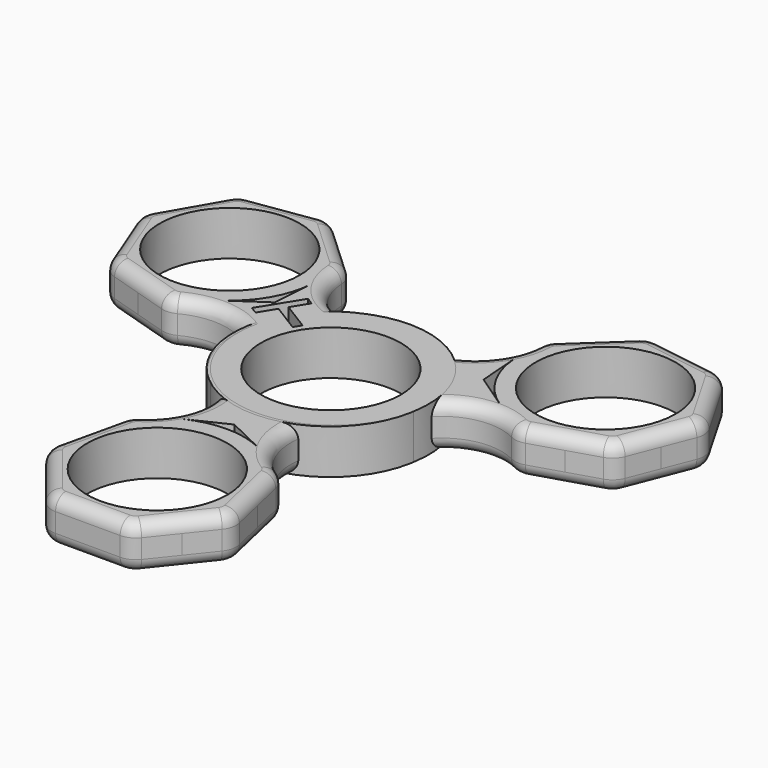
from build123d import *

# Parameters (mm, degrees)
F1_DEPTH       = 7
F2_R           = 10.9982
F3_DEPTH       = 7.001
F5_COUNT       = 3
F6_R           = 3.1
F6_2_R         = 3.1
F6_3_R         = 3.1
F7_T1_DEPTH    = 10.2686412317
F7_T3_DEPTH    = 10.25929714
F7_T5_DEPTH    = 10.1415011295
F7_T7_DEPTH    = 10.1415011295
F7_T9_DEPTH    = 10.1415011295
F7_T12_ANGLE   = 51.4285714286
F7_T14_ANGLE   = 44.6985802325
F7_T18_ANGLE   = 95.7149736929
F7_S19_R       = 15.0569162084
F7_T20_DEPTH   = 12
F7_T22_ANGLE   = 51.4285714286
F7_T24_ANGLE   = 51.4285714286
F7_T26_ANGLE   = 51.4285714286
F7_T28_ANGLE   = 44.1929451945
F7_T32_ANGLE   = 104.4319543532
F7_S33_R       = 15.0569162084
F7_T34_DEPTH   = 13
F7_T36_ANGLE   = 44.1929451945
F7_T38_ANGLE   = 51.4285714286
F7_T40_ANGLE   = 51.4285714286
F7_T42_ANGLE   = 51.4285714286
F7_T44_ANGLE   = 51.4285714286
F7_T46_ANGLE   = 44.6985802325
F7_T50_ANGLE   = 95.7149736929
F7_S51_R       = 15.0569162084
F7_T52_DEPTH   = 12
F7_T56_ANGLE   = 104.4319543532
F7_S57_R       = 15.0569162084
F7_T58_DEPTH   = 13
F7_2_T1_DEPTH  = 10.1415011295
F7_2_T3_DEPTH  = 10.2686412317
F7_2_T5_DEPTH  = 10.1415011295
F7_2_T7_DEPTH  = 10.1415011295
F7_2_T9_DEPTH  = 10.25929714
F7_2_T12_ANGLE = 44.1929451945
F7_2_T14_ANGLE = 51.4285714286
F7_2_T16_ANGLE = 51.4285714286
F7_2_T18_ANGLE = 51.4285714286
F7_2_T20_ANGLE = 51.4285714286
F7_2_T22_ANGLE = 44.6985802325
F7_2_T26_ANGLE = 95.7149736929
F7_2_S27_R     = 15.0569162084
F7_2_T28_DEPTH = 13
F7_2_T32_ANGLE = 104.4319543532
F7_2_S33_R     = 15.0569162084
F7_2_T34_DEPTH = 12
F7_2_T36_ANGLE = 51.4285714286
F7_2_T38_ANGLE = 51.4285714286
F7_2_T40_ANGLE = 44.6985802325
F7_2_T44_ANGLE = 95.7149736929
F7_2_S45_R     = 15.0569162084
F7_2_T46_DEPTH = 13
F7_2_T48_ANGLE = 51.4285714286
F7_2_T50_ANGLE = 51.4285714286
F7_2_T52_ANGLE = 44.1929451945
F7_2_T56_ANGLE = 104.4319543532
F7_2_S57_R     = 15.0569162084
F7_2_T58_DEPTH = 12
F7_3_T1_DEPTH  = 10.25929714
F7_3_T3_DEPTH  = 10.1415011295
F7_3_T5_DEPTH  = 10.1415011295
F7_3_T7_DEPTH  = 10.1415011295
F7_3_T9_DEPTH  = 10.2686412317
F7_3_T12_ANGLE = 44.1929451945
F7_3_T14_ANGLE = 51.4285714286
F7_3_T16_ANGLE = 51.4285714286
F7_3_T18_ANGLE = 51.4285714286
F7_3_T20_ANGLE = 51.4285714286
F7_3_T22_ANGLE = 44.6985802325
F7_3_T26_ANGLE = 95.7149736929
F7_3_S27_R     = 15.0569162084
F7_3_T28_DEPTH = 13
F7_3_T32_ANGLE = 104.4319543532
F7_3_S33_R     = 15.0569162084
F7_3_T34_DEPTH = 13
F7_3_T36_ANGLE = 51.4285714286
F7_3_T38_ANGLE = 51.4285714286
F7_3_T40_ANGLE = 44.1929451945
F7_3_T44_ANGLE = 104.4319543532
F7_3_S45_R     = 15.0569162084
F7_3_T46_DEPTH = 13
F7_3_T48_ANGLE = 51.4285714286
F7_3_T50_ANGLE = 51.4285714286
F7_3_T52_ANGLE = 44.6985802325
F7_3_T56_ANGLE = 95.7149736929
F7_3_S57_R     = 15.0569162084
F7_3_T58_DEPTH = 13
F8_R           = 10.9982
F9_DEPTH       = 7.0010001


# Not quite as in the source:
# - a fillet or chamfer that OpenCascade refuses, or shapes differently, is made with other operations: its cross-section is extruded or revolved along the edge and cut away or added
# - a feature names something its author has since deleted; it is built from what else it names


with BuildPart() as f1:
    # F0 (on Top) → F1 (new body)
    with BuildSketch(Plane.XY):
        with BuildLine():
            ThreePointArc((10.6559893288, -42.5716732307), (12.8646786322, -38.5753509396), (13.6295220444, -34.0738051109))
            ThreePointArc((13.6295220444, -34.0738051109), (13.5438224971, -32.5477830518), (13.2878015765, -31.0409515996))
            ThreePointArc((13.2878015765, -31.0409515996), (10.655989621, -25.5759373575), (5.9136281245, -21.7940301308))
            ThreePointArc((5.9136281245, -21.7940301308), (-6.034e-07, -20.4442830665), (-5.9136292117, -21.7940306543))
            ThreePointArc((-5.9136292117, -21.7940306543), (-10.655989762, -25.5759375342), (-13.2878014086, -31.0409508638))
            ThreePointArc((-13.2878014086, -31.0409508638), (-13.28780149, -37.1066590013), (-10.6559893588, -42.5716731931))
            ThreePointArc((-10.6559893588, -42.5716731931), (-5.9136279392, -46.3535801803), (-4e-10, -47.7033271552))
            ThreePointArc((-4e-10, -47.7033271552), (5.9136279171, -46.3535801909), (10.6559893288, -42.5716732307))
        make_face()
        with BuildLine():
            ThreePointArc((13.2878015765, -31.0409515996), (13.5438224971, -32.5477830518), (13.6295220444, -34.0738051109))
            ThreePointArc((13.6295220444, -34.0738051109), (12.8646786322, -38.5753509396), (10.6559893288, -42.5716732307))
            Line((10.6559893288, -42.5716732307), (14.7483469675, -37.4400190643))
            Line((14.7483469675, -37.4400190643), (13.2878015765, -31.0409515996))
        make_face()
        with BuildLine():
            ThreePointArc((5.9136281245, -21.7940301308), (10.655989621, -25.5759373575), (13.2878015765, -31.0409515996))
            Line((13.2878015765, -31.0409515996), (11.827255974, -24.6418832081))
            Line((11.827255974, -24.6418832081), (6.1794303068, -21.9220337154))
            Line((6.1794303068, -21.9220337154), (5.9136281245, -21.7940301308))
        make_face()
        with BuildLine():
            Line((6.563631883, -47.7033271552), (10.6559893288, -42.5716732307))
            ThreePointArc((10.6559893288, -42.5716732307), (5.9136279171, -46.3535801909), (-4e-10, -47.7033271552))
            Line((-4e-10, -47.7033271552), (6.563631883, -47.7033271552))
        make_face()
        with BuildLine():
            Line((0, -18.9461769209), (5.9136281245, -21.7940301308))
            Line((5.9136281245, -21.7940301308), (6.1794303068, -21.9220337154))
            ThreePointArc((6.1794303068, -21.9220337154), (4.8033446668, -17.8576663017), (4.8404350008, -13.5668250708))
            Line((4.8404350008, -13.5668250708), (6.1794303068, -13.5668250708))
            ThreePointArc((6.1794303068, -13.5668250708), (-0.1592409852, 15.0955047693), (-6.9180878725, -13.4706621833))
            Line((-6.9180878725, -13.4706621833), (-5.5738588853, -13.4706621833))
            ThreePointArc((-5.5738588853, -13.4706621833), (-5.5961038295, -18.7704883426), (-8.6417702198, -23.1078341203))
            Line((-8.6417702198, -23.1078341203), (-5.9136292117, -21.7940306543))
            Line((-5.9136292117, -21.7940306543), (0, -18.9461769209))
        make_face()
        with BuildLine():
            Line((6.1794303068, -21.9220337154), (11.827255974, -24.6418832081))
            ThreePointArc((11.827255974, -24.6418832081), (7.1362076022, -20.0565167273), (6.1794303068, -13.5668250708))
            Line((6.1794303068, -13.5668250708), (4.8404350008, -13.5668250708))
            ThreePointArc((4.8404350008, -13.5668250708), (4.8033446668, -17.8576663017), (6.1794303068, -21.9220337154))
        make_face()
        with BuildLine():
            Line((-6.563631883, -47.7033271552), (-4e-10, -47.7033271552))
            ThreePointArc((-4e-10, -47.7033271552), (-5.9136279392, -46.3535801803), (-10.6559893588, -42.5716731931))
            Line((-10.6559893588, -42.5716731931), (-6.563631883, -47.7033271552))
        make_face()
        with BuildLine():
            ThreePointArc((-13.2878014086, -31.0409508638), (-10.655989762, -25.5759375342), (-5.9136292117, -21.7940306543))
            Line((-5.9136292117, -21.7940306543), (-8.6417702198, -23.1078341203))
            Line((-8.6417702198, -23.1078341203), (-11.827255974, -24.6418832081))
            Line((-11.827255974, -24.6418832081), (-13.2878014086, -31.0409508638))
        make_face()
        with BuildLine():
            Line((-14.7483469675, -37.4400190643), (-10.6559893588, -42.5716731931))
            ThreePointArc((-10.6559893588, -42.5716731931), (-13.28780149, -37.1066590013), (-13.2878014086, -31.0409508638))
            Line((-13.2878014086, -31.0409508638), (-14.7483469675, -37.4400190643))
        make_face()
        with BuildLine():
            Line((-11.827255974, -24.6418832081), (-8.6417702198, -23.1078341203))
            ThreePointArc((-8.6417702198, -23.1078341203), (-5.5961038295, -18.7704883426), (-5.5738588853, -13.4706621833))
            Line((-5.5738588853, -13.4706621833), (-6.9180878725, -13.4706621833))
            ThreePointArc((-6.9180878725, -13.4706621833), (-7.3085566508, -19.963343537), (-11.827255974, -24.6418832081))
        make_face()
    extrude(amount=F1_DEPTH)

    # F2 (on face) → F3 (cut, through all)
    with BuildSketch(Plane.XY.offset(7)):
        Circle(F2_R)
        with Locations((0, -34.0738051109)):
            Circle(F2_R)
    extrude(amount=-F3_DEPTH, mode=Mode.SUBTRACT)


with BuildPart() as f5_1:
    # F5: instance of F1
    add(f1.part.rotate(Axis((0, 0, 10.0436238572), (0, 0, 1)), 1 * 360 / F5_COUNT))

    # F6#2
    f6_2_edges = [f5_1.edges().sort_by_distance(p)[0] for p in [
        (15.426869, 22.563646, 3.5),
        (25.049834, 31.492453, 3.5),
        (38.030477, 29.535936, 3.5),
        (44.594109, 18.167392, 3.5),
        (39.798181, 5.947566, 3.5),
        (27.254125, 2.078237, 3.5),
    ]]
    fillet(f6_2_edges, radius=F6_2_R)

    # F7#2: fillet of radius 2 on 2 edges, made by hand

    # F7_2_s2 → F7_2_t1 (cut)
    with BuildSketch(Plane(origin=(31.3565415396, -4.7262381861, 0), x_dir=(0, 0, 1), z_dir=(-0.9888308262, 0.1490422662, 0))):
        with BuildLine():
            ThreePointArc((7, 32.8741920415), (6.4142135624, 34.2884056039), (5, 34.8741920415))
            Line((5, 34.8741920415), (7, 34.8741920415))
            Line((7, 34.8741920415), (7, 32.8741920415))
        make_face()
        with BuildLine():
            ThreePointArc((0, 32.8741920415), (0.5857864376, 34.2884056039), (2, 34.8741920415))
            Line((2, 34.8741920415), (0, 34.8741920415))
            Line((0, 34.8741920415), (0, 32.8741920415))
        make_face()
    extrude(amount=F7_2_T1_DEPTH, mode=Mode.SUBTRACT)

    # F7_2_s4 → F7_2_t3 (cut)
    with BuildSketch(Plane(origin=(26.7766913665, 8.25951543, 0), x_dir=(0, 0, 1), z_dir=(0.9555728058, 0.2947551744, 0))):
        with BuildLine():
            ThreePointArc((2, 6.0473871076), (0.5857864376, 5.46160067), (0, 4.0473871076))
            Line((0, 4.0473871076), (0, 6.0473871076))
            Line((0, 6.0473871076), (2, 6.0473871076))
        make_face()
        with BuildLine():
            ThreePointArc((5, 6.0473871076), (6.4142135624, 5.46160067), (7, 4.0473871076))
            Line((7, 4.0473871076), (7, 6.0473871076))
            Line((7, 6.0473871076), (5, 6.0473871076))
        make_face()
    extrude(amount=F7_2_T3_DEPTH, mode=Mode.SUBTRACT)

    # F7_2_s6 → F7_2_t5 (cut)
    with BuildSketch(Plane(origin=(7.880122025, 20.0782234679, 0), x_dir=(0, 0, 1), z_dir=(0.3653410244, 0.9308737486, 0))):
        with BuildLine():
            ThreePointArc((0, 32.8741920415), (0.5857864376, 34.2884056039), (2, 34.8741920415))
            Line((2, 34.8741920415), (0, 34.8741920415))
            Line((0, 34.8741920415), (0, 32.8741920415))
        make_face()
        with BuildLine():
            ThreePointArc((7, 32.8741920415), (6.4142135624, 34.2884056039), (5, 34.8741920415))
            Line((5, 34.8741920415), (7, 34.8741920415))
            Line((7, 34.8741920415), (7, 32.8741920415))
        make_face()
    extrude(amount=F7_2_T5_DEPTH, mode=Mode.SUBTRACT)

    # F7_2_s8 → F7_2_t7 (cut)
    with BuildSketch(Plane(origin=(2.5353752824, -4.3913988053, 0), x_dir=(0, 0, 1), z_dir=(-0.5, 0.8660254038, 0))):
        with BuildLine():
            ThreePointArc((0, 45.7033271552), (0.5857864376, 47.1175407176), (2, 47.7033271552))
            Line((2, 47.7033271552), (0, 47.7033271552))
            Line((0, 47.7033271552), (0, 45.7033271552))
        make_face()
        with BuildLine():
            ThreePointArc((7, 45.7033271552), (6.4142135624, 47.1175407176), (5, 47.7033271552))
            Line((5, 47.7033271552), (7, 47.7033271552))
            Line((7, 47.7033271552), (7, 45.7033271552))
        make_face()
    extrude(amount=F7_2_T7_DEPTH, mode=Mode.SUBTRACT)

    # F7_2_s10 → F7_2_t9 (cut)
    with BuildSketch(Plane(origin=(28.0687425446, 26.0439870574, 0), x_dir=(0, 0, 1), z_dir=(-0.7330518718, -0.6801727378, 0))):
        with BuildLine():
            ThreePointArc((0, 4.0473871076), (0.5857864376, 5.46160067), (2, 6.0473871076))
            Line((2, 6.0473871076), (0, 6.0473871076))
            Line((0, 6.0473871076), (0, 4.0473871076))
        make_face()
        with BuildLine():
            ThreePointArc((7, 4.0473871076), (6.4142135624, 5.46160067), (5, 6.0473871076))
            Line((5, 6.0473871076), (7, 6.0473871076))
            Line((7, 6.0473871076), (7, 4.0473871076))
        make_face()
    extrude(amount=F7_2_T9_DEPTH, mode=Mode.SUBTRACT)

    # F7_2_s11 → F7_2_t12 (revolve, cut)
    with BuildSketch(Plane(origin=(26.7766913665, 8.25951543, 0), x_dir=(0, 0, 1), z_dir=(0.9555728058, 0.2947551744, 0))):
        with BuildLine():
            ThreePointArc((0, 4.0473871076), (0.5857864376, 5.46160067), (2, 6.0473871076))
            Line((2, 6.0473871076), (0, 6.0473871076))
            Line((0, 6.0473871076), (0, 4.0473871076))
        make_face()
    revolve(axis=Axis((27.6454489675, 5.4430724618, 0), (0, 0, -1)), revolution_arc=F7_2_T12_ANGLE, mode=Mode.SUBTRACT)

    # F7_2_s13 → F7_2_t14 (revolve, cut)
    with BuildSketch(Plane(origin=(36.5891256799, 11.2862505672, 0), x_dir=(0, 0, 1), z_dir=(-0.9555728058, -0.2947551744, 0))):
        with BuildLine():
            ThreePointArc((0, -4.0473871076), (0.5857864376, -5.46160067), (2, -6.0473871076))
            Line((2, -6.0473871076), (0, -6.0473871076))
            Line((0, -6.0473871076), (0, -4.0473871076))
        make_face()
    revolve(axis=Axis((37.4578832809, 8.469807599, 0), (0, 0, 1)), revolution_arc=F7_2_T14_ANGLE, mode=Mode.SUBTRACT)

    # F7_2_s15 → F7_2_t16 (revolve, cut)
    with BuildSketch(Plane(origin=(11.5852284363, 29.5186806412, 0), x_dir=(0, 0, 1), z_dir=(-0.3653410244, -0.9308737486, 0))):
        with BuildLine():
            ThreePointArc((0, -32.8741920415), (0.5857864376, -34.2884056039), (2, -34.8741920415))
            Line((2, -34.8741920415), (0, -34.8741920415))
            Line((0, -34.8741920415), (0, -32.8741920415))
        make_face()
    revolve(axis=Axis((41.1629896921, 17.9102647723, 0), (0, 0, 1)), revolution_arc=F7_2_T16_ANGLE, mode=Mode.SUBTRACT)

    # F7_2_s17 → F7_2_t18 (revolve, cut)
    with BuildSketch(Plane(origin=(-2.5353752824, 4.3913988053, 0), x_dir=(0, 0, 1), z_dir=(0.5, -0.8660254038, 0))):
        with BuildLine():
            ThreePointArc((0, -45.7033271552), (0.5857864376, -47.1175407176), (2, -47.7033271552))
            Line((2, -47.7033271552), (0, -47.7033271552))
            Line((0, -47.7033271552), (0, -45.7033271552))
        make_face()
    revolve(axis=Axis((36.0922391274, 26.6930623829, 0), (0, 0, 1)), revolution_arc=F7_2_T18_ANGLE, mode=Mode.SUBTRACT)

    # F7_2_s19 → F7_2_t20 (revolve, cut)
    with BuildSketch(Plane(origin=(21.3283125986, -3.2147258753, 0), x_dir=(0, 0, 1), z_dir=(0.9888308262, -0.1490422662, 0))):
        with BuildLine():
            ThreePointArc((0, -32.8741920415), (0.5857864376, -34.2884056039), (2, -34.8741920415))
            Line((2, -34.8741920415), (0, -34.8741920415))
            Line((0, -34.8741920415), (0, -32.8741920415))
        make_face()
    revolve(axis=Axis((26.0640101864, 28.2045746937, 0), (0, 0, 1)), revolution_arc=F7_2_T20_ANGLE, mode=Mode.SUBTRACT)

    # F7_2_s21 → F7_2_t22 (revolve, cut)
    with BuildSketch(Plane(origin=(0.9381651249, 21.9779882774, 0), x_dir=(0, 0, 1), z_dir=(-0.0426477412, -0.9990901712, 0))):
        with BuildLine():
            ThreePointArc((0, -16.5212804378), (0.5857864376, -15.1070668755), (2, -14.5212804378))
            Line((2, -14.5212804378), (0, -14.5212804378))
            Line((0, -14.5212804378), (0, -16.5212804378))
        make_face()
    revolve(axis=Axis((18.5434132142, 21.2264804704, 0), (0, 0, -1)), revolution_arc=F7_2_T22_ANGLE, mode=Mode.SUBTRACT)


with BuildPart() as f5_2:
    # F5: instance of F1
    add(f1.part.rotate(Axis((0, 0, 10.0436238572), (0, 0, 1)), 2 * 360 / F5_COUNT))

    # F6
    f6_edges = [f5_2.edges().sort_by_distance(p)[0] for p in [
        (-44.594109, 18.167392, 3.5),
        (-38.030477, 29.535936, 3.5),
        (-25.049834, 31.492453, 3.5),
        (-39.798181, 5.947566, 3.5),
        (-27.254125, 2.078237, 3.5),
        (-15.426869, 22.563646, 3.5),
    ]]
    fillet(f6_edges, radius=F6_R)

    # F7: fillet of radius 2 on 2 edges, made by hand

    # F7_s2 → F7_t1 (cut)
    with BuildSketch(Plane(origin=(-20.5412958686, 19.0595372377, 0), x_dir=(0, 0, 1), z_dir=(-0.7330518718, 0.6801727378, 0))):
        with BuildLine():
            ThreePointArc((5, 6.0473871076), (6.4142135624, 5.46160067), (7, 4.0473871076))
            Line((7, 4.0473871076), (7, 6.0473871076))
            Line((7, 6.0473871076), (5, 6.0473871076))
        make_face()
        with BuildLine():
            ThreePointArc((2, 6.0473871076), (0.5857864376, 5.46160067), (0, 4.0473871076))
            Line((0, 4.0473871076), (0, 6.0473871076))
            Line((0, 6.0473871076), (2, 6.0473871076))
        make_face()
    extrude(amount=F7_T1_DEPTH, mode=Mode.SUBTRACT)

    # F7_s4 → F7_t3 (cut)
    with BuildSketch(Plane(origin=(-36.5891256799, 11.2862505672, 0), x_dir=(0, 0, 1), z_dir=(0.9555728058, -0.2947551744, 0))):
        with BuildLine():
            ThreePointArc((0, 4.0473871076), (0.5857864376, 5.46160067), (2, 6.0473871076))
            Line((2, 6.0473871076), (0, 6.0473871076))
            Line((0, 6.0473871076), (0, 4.0473871076))
        make_face()
        with BuildLine():
            ThreePointArc((7, 4.0473871076), (6.4142135624, 5.46160067), (5, 6.0473871076))
            Line((5, 6.0473871076), (7, 6.0473871076))
            Line((7, 6.0473871076), (7, 4.0473871076))
        make_face()
    extrude(amount=F7_T3_DEPTH, mode=Mode.SUBTRACT)

    # F7_s6 → F7_t5 (cut)
    with BuildSketch(Plane(origin=(-11.5852284363, 29.5186806412, 0), x_dir=(0, 0, 1), z_dir=(0.3653410244, -0.9308737486, 0))):
        with BuildLine():
            ThreePointArc((0, 32.8741920415), (0.5857864376, 34.2884056039), (2, 34.8741920415))
            Line((2, 34.8741920415), (0, 34.8741920415))
            Line((0, 34.8741920415), (0, 32.8741920415))
        make_face()
        with BuildLine():
            ThreePointArc((7, 32.8741920415), (6.4142135624, 34.2884056039), (5, 34.8741920415))
            Line((5, 34.8741920415), (7, 34.8741920415))
            Line((7, 34.8741920415), (7, 32.8741920415))
        make_face()
    extrude(amount=F7_T5_DEPTH, mode=Mode.SUBTRACT)

    # F7_s8 → F7_t7 (cut)
    with BuildSketch(Plane(origin=(2.5353752824, 4.3913988053, 0), x_dir=(0, 0, 1), z_dir=(-0.5, -0.8660254038, 0))):
        with BuildLine():
            ThreePointArc((0, 45.7033271552), (0.5857864376, 47.1175407176), (2, 47.7033271552))
            Line((2, 47.7033271552), (0, 47.7033271552))
            Line((0, 47.7033271552), (0, 45.7033271552))
        make_face()
        with BuildLine():
            ThreePointArc((7, 45.7033271552), (6.4142135624, 47.1175407176), (5, 47.7033271552))
            Line((5, 47.7033271552), (7, 47.7033271552))
            Line((7, 47.7033271552), (7, 45.7033271552))
        make_face()
    extrude(amount=F7_T7_DEPTH, mode=Mode.SUBTRACT)

    # F7_s10 → F7_t9 (cut)
    with BuildSketch(Plane(origin=(-21.3283125986, -3.2147258753, 0), x_dir=(0, 0, 1), z_dir=(-0.9888308262, -0.1490422662, 0))):
        with BuildLine():
            ThreePointArc((0, 32.8741920415), (0.5857864376, 34.2884056039), (2, 34.8741920415))
            Line((2, 34.8741920415), (0, 34.8741920415))
            Line((0, 34.8741920415), (0, 32.8741920415))
        make_face()
        with BuildLine():
            ThreePointArc((7, 32.8741920415), (6.4142135624, 34.2884056039), (5, 34.8741920415))
            Line((5, 34.8741920415), (7, 34.8741920415))
            Line((7, 34.8741920415), (7, 32.8741920415))
        make_face()
    extrude(amount=F7_T9_DEPTH, mode=Mode.SUBTRACT)

    # F7_s11 → F7_t12 (revolve, cut)
    with BuildSketch(Plane(origin=(-7.880122025, 20.0782234679, 0), x_dir=(0, 0, 1), z_dir=(-0.3653410244, 0.9308737486, 0))):
        with BuildLine():
            ThreePointArc((0, -32.8741920415), (0.5857864376, -34.2884056039), (2, -34.8741920415))
            Line((2, -34.8741920415), (0, -34.8741920415))
            Line((0, -34.8741920415), (0, -32.8741920415))
        make_face()
    revolve(axis=Axis((-37.4578832809, 8.469807599, 0), (0, 0, 1)), revolution_arc=F7_T12_ANGLE, mode=Mode.SUBTRACT)

    # F7_s13 → F7_t14 (revolve, cut)
    with BuildSketch(Plane(origin=(-19.5025787348, -10.1765193076, 0), x_dir=(0, 0, 1), z_dir=(0.8865613395, 0.4626110583, 0))):
        with BuildLine():
            ThreePointArc((0, -16.5212804378), (0.5857864376, -15.1070668755), (2, -14.5212804378))
            Line((2, -14.5212804378), (0, -14.5212804378))
            Line((0, -14.5212804378), (0, -16.5212804378))
        make_face()
    revolve(axis=Axis((-27.6543779274, 5.4458266812, 0), (0, 0, -1)), revolution_arc=F7_T14_ANGLE, mode=Mode.SUBTRACT)


with BuildPart() as f1_1:
    add(f1.part)

    # F6#3
    f6_3_edges = [f1_1.edges().sort_by_distance(p)[0] for p in [
        (11.827256, -24.641883, 3.5),
        (14.748347, -37.440019, 3.5),
        (6.563632, -47.703327, 3.5),
        (-6.563632, -47.703327, 3.5),
        (-14.748347, -37.440019, 3.5),
        (-11.827256, -24.641883, 3.5),
    ]]
    fillet(f6_3_edges, radius=F6_3_R)

    # F7#3: fillet of radius 2 on 5 edges, made by hand

    # F7_3_s2 → F7_3_t1 (cut)
    with BuildSketch(Plane(origin=(8.5203831353, -37.3302376247, 0), x_dir=(0, 0, 1), z_dir=(-0.222520934, 0.9749279122, 0))):
        with BuildLine():
            ThreePointArc((0, 4.0473871076), (0.5857864376, 5.46160067), (2, 6.0473871076))
            Line((2, 6.0473871076), (0, 6.0473871076))
            Line((0, 6.0473871076), (0, 4.0473871076))
        make_face()
        with BuildLine():
            ThreePointArc((7, 4.0473871076), (6.4142135624, 5.46160067), (5, 6.0473871076))
            Line((5, 6.0473871076), (7, 6.0473871076))
            Line((7, 6.0473871076), (7, 4.0473871076))
        make_face()
    extrude(amount=F7_3_T1_DEPTH, mode=Mode.SUBTRACT)

    # F7_3_s4 → F7_3_t3 (cut)
    with BuildSketch(Plane(origin=(-19.7713131033, -24.7924424551, 0), x_dir=(0, 0, 1), z_dir=(0.6234898019, 0.7818314825, 0))):
        with BuildLine():
            ThreePointArc((0, 32.8741920415), (0.5857864376, 34.2884056039), (2, 34.8741920415))
            Line((2, 34.8741920415), (0, 34.8741920415))
            Line((0, 34.8741920415), (0, 32.8741920415))
        make_face()
        with BuildLine():
            ThreePointArc((7, 32.8741920415), (6.4142135624, 34.2884056039), (5, 34.8741920415))
            Line((5, 34.8741920415), (7, 34.8741920415))
            Line((7, 34.8741920415), (7, 32.8741920415))
        make_face()
    extrude(amount=F7_3_T3_DEPTH, mode=Mode.SUBTRACT)

    # F7_3_s6 → F7_3_t5 (cut)
    with BuildSketch(Plane.YZ.offset(-5.0707505647)):
        with BuildLine():
            ThreePointArc((-45.7033271552, 0), (-47.1175407176, 0.5857864376), (-47.7033271552, 2))
            Line((-47.7033271552, 2), (-47.7033271552, 0))
            Line((-47.7033271552, 0), (-45.7033271552, 0))
        make_face()
        with BuildLine():
            ThreePointArc((-45.7033271552, 7), (-47.1175407176, 6.4142135624), (-47.7033271552, 5))
            Line((-47.7033271552, 5), (-47.7033271552, 7))
            Line((-47.7033271552, 7), (-45.7033271552, 7))
        make_face()
    extrude(amount=F7_3_T5_DEPTH, mode=Mode.SUBTRACT)

    # F7_3_s8 → F7_3_t7 (cut)
    with BuildSketch(Plane(origin=(13.4481905735, -16.8634975926, 0), x_dir=(0, 0, 1), z_dir=(0.6234898019, -0.7818314825, 0))):
        with BuildLine():
            ThreePointArc((0, 32.8741920415), (0.5857864376, 34.2884056039), (2, 34.8741920415))
            Line((2, 34.8741920415), (0, 34.8741920415))
            Line((0, 34.8741920415), (0, 32.8741920415))
        make_face()
        with BuildLine():
            ThreePointArc((7, 32.8741920415), (6.4142135624, 34.2884056039), (5, 34.8741920415))
            Line((5, 34.8741920415), (7, 34.8741920415))
            Line((7, 34.8741920415), (7, 32.8741920415))
        make_face()
    extrude(amount=F7_3_T7_DEPTH, mode=Mode.SUBTRACT)

    # F7_3_s10 → F7_3_t9 (cut)
    with BuildSketch(Plane(origin=(-6.2353954979, -27.3190526677, 0), x_dir=(0, 0, 1), z_dir=(-0.222520934, -0.9749279122, 0))):
        with BuildLine():
            ThreePointArc((5, 6.0473871076), (6.4142135624, 5.46160067), (7, 4.0473871076))
            Line((7, 4.0473871076), (7, 6.0473871076))
            Line((7, 6.0473871076), (5, 6.0473871076))
        make_face()
        with BuildLine():
            ThreePointArc((2, 6.0473871076), (0.5857864376, 5.46160067), (0, 4.0473871076))
            Line((0, 4.0473871076), (0, 6.0473871076))
            Line((0, 6.0473871076), (2, 6.0473871076))
        make_face()
    extrude(amount=F7_3_T9_DEPTH, mode=Mode.SUBTRACT)

    # F7_3_s11 → F7_3_t12 (revolve, cut)
    with BuildSketch(Plane(origin=(-6.2353954979, -27.3190526677, 0), x_dir=(0, 0, 1), z_dir=(-0.222520934, -0.9749279122, 0))):
        with BuildLine():
            ThreePointArc((5, 6.0473871076), (6.4142135624, 5.46160067), (7, 4.0473871076))
            Line((7, 4.0473871076), (7, 6.0473871076))
            Line((7, 6.0473871076), (5, 6.0473871076))
        make_face()
    revolve(axis=Axis((-9.1088854572, -26.6631973358, 7), (0, 0, -1)), revolution_arc=F7_3_T12_ANGLE, mode=Mode.SUBTRACT)

    # F7_3_s13 → F7_3_t14 (revolve, cut)
    with BuildSketch(Plane(origin=(-8.5203831353, -37.3302376247, 0), x_dir=(0, 0, 1), z_dir=(0.222520934, 0.9749279122, 0))):
        with BuildLine():
            ThreePointArc((5, -6.0473871076), (6.4142135624, -5.46160067), (7, -4.0473871076))
            Line((7, -4.0473871076), (7, -6.0473871076))
            Line((7, -6.0473871076), (5, -6.0473871076))
        make_face()
    revolve(axis=Axis((-11.3938730945, -36.6743822927, 7), (0, 0, 1)), revolution_arc=F7_3_T14_ANGLE, mode=Mode.SUBTRACT)

    # F7_3_s15 → F7_3_t16 (revolve, cut)
    with BuildSketch(Plane(origin=(19.7713131033, -24.7924424551, 0), x_dir=(0, 0, 1), z_dir=(-0.6234898019, 0.7818314825, 0))):
        with BuildLine():
            ThreePointArc((7, -32.8741920415), (6.4142135624, -34.2884056039), (5, -34.8741920415))
            Line((5, -34.8741920415), (7, -34.8741920415))
            Line((7, -34.8741920415), (7, -32.8741920415))
        make_face()
    revolve(axis=Axis((-5.0707505647, -44.6033271552, 7), (0, 0, 1)), revolution_arc=F7_3_T16_ANGLE, mode=Mode.SUBTRACT)

    # F7_3_s17 → F7_3_t18 (revolve, cut)
    with BuildSketch(Plane.YZ.offset(5.0707505647)):
        with BuildLine():
            ThreePointArc((-45.7033271552, 7), (-47.1175407176, 6.4142135624), (-47.7033271552, 5))
            Line((-47.7033271552, 5), (-47.7033271552, 7))
            Line((-47.7033271552, 7), (-45.7033271552, 7))
        make_face()
    revolve(axis=Axis((5.0707505647, -44.6033271552, 7), (0, 0, 1)), revolution_arc=F7_3_T18_ANGLE, mode=Mode.SUBTRACT)

    # F7_3_s19 → F7_3_t20 (revolve, cut)
    with BuildSketch(Plane(origin=(-13.4481905735, -16.8634975926, 0), x_dir=(0, 0, 1), z_dir=(-0.6234898019, -0.7818314825, 0))):
        with BuildLine():
            ThreePointArc((7, -32.8741920415), (6.4142135624, -34.2884056039), (5, -34.8741920415))
            Line((5, -34.8741920415), (7, -34.8741920415))
            Line((7, -34.8741920415), (7, -32.8741920415))
        make_face()
    revolve(axis=Axis((11.3938730945, -36.6743822927, 7), (0, 0, 1)), revolution_arc=F7_3_T20_ANGLE, mode=Mode.SUBTRACT)

    # F7_3_s21 → F7_3_t22 (revolve, cut)
    with BuildSketch(Plane(origin=(18.5644136098, -11.8014689698, 0), x_dir=(0, 0, 1), z_dir=(-0.8439135983, 0.5364791129, 0))):
        with BuildLine():
            ThreePointArc((7, -16.5212804378), (6.4142135624, -15.1070668755), (5, -14.5212804378))
            Line((5, -14.5212804378), (7, -14.5212804378))
            Line((7, -14.5212804378), (7, -16.5212804378))
        make_face()
    revolve(axis=Axis((9.1109647132, -26.6723071515, 7), (0, 0, -1)), revolution_arc=F7_3_T22_ANGLE, mode=Mode.SUBTRACT)


with BuildPart() as f7_tool16:
    # F7_s17 → F7_t18 (revolve)
    with BuildSketch(Plane(origin=(-19.5025787348, -10.1765193076, 0), x_dir=(0, 0, 1), z_dir=(-0.8865613395, -0.4626110583, 0))):
        with BuildLine():
            ThreePointArc((0, 16.5212804378), (0.5857864376, 15.1070668755), (2, 14.5212804378))
            Line((2, 14.5212804378), (0, 14.5212804378))
            Line((0, 14.5212804378), (0, 16.5212804378))
        make_face()
    revolve(axis=Axis((-21.4712902989, -6.4036229837, 0), (0, 0, -1)), revolution_arc=F7_T18_ANGLE)

    # F7_s19 → F7_t20 (cut, symmetric)
    with BuildSketch(Plane.XY.offset(1.7)):
        with Locations((0.1686635827, 0.2141451478)):
            Circle(F7_S19_R)
    extrude(amount=F7_T20_DEPTH, both=True, mode=Mode.SUBTRACT)


with BuildPart() as f5_2_1:
    add(f5_2.part)

    # F7_t15: cut F7_tool16
    add(f7_tool16.part, mode=Mode.SUBTRACT)

    # F7_s21 → F7_t22 (revolve, cut)
    with BuildSketch(Plane(origin=(-2.5353752824, -4.3913988053, 0), x_dir=(0, 0, 1), z_dir=(0.5, 0.8660254038, 0))):
        with BuildLine():
            ThreePointArc((0, -45.7033271552), (0.5857864376, -47.1175407176), (2, -47.7033271552))
            Line((2, -47.7033271552), (0, -47.7033271552))
            Line((0, -47.7033271552), (0, -45.7033271552))
        make_face()
    revolve(axis=Axis((-41.1629896921, 17.9102647723, 0), (0, 0, 1)), revolution_arc=F7_T22_ANGLE, mode=Mode.SUBTRACT)

    # F7_s23 → F7_t24 (revolve, cut)
    with BuildSketch(Plane(origin=(-31.3565415396, -4.7262381861, 0), x_dir=(0, 0, 1), z_dir=(0.9888308262, 0.1490422662, 0))):
        with BuildLine():
            ThreePointArc((0, -32.8741920415), (0.5857864376, -34.2884056039), (2, -34.8741920415))
            Line((2, -34.8741920415), (0, -34.8741920415))
            Line((0, -34.8741920415), (0, -32.8741920415))
        make_face()
    revolve(axis=Axis((-36.0922391274, 26.6930623829, 0), (0, 0, 1)), revolution_arc=F7_T24_ANGLE, mode=Mode.SUBTRACT)

    # F7_s25 → F7_t26 (revolve, cut)
    with BuildSketch(Plane(origin=(-28.0687425446, 26.0439870574, 0), x_dir=(0, 0, 1), z_dir=(0.7330518718, -0.6801727378, 0))):
        with BuildLine():
            ThreePointArc((0, -4.0473871076), (0.5857864376, -5.46160067), (2, -6.0473871076))
            Line((2, -6.0473871076), (0, -6.0473871076))
            Line((0, -6.0473871076), (0, -4.0473871076))
        make_face()
    revolve(axis=Axis((-26.0640101864, 28.2045746937, 0), (0, 0, 1)), revolution_arc=F7_T26_ANGLE, mode=Mode.SUBTRACT)

    # F7_s27 → F7_t28 (revolve, cut)
    with BuildSketch(Plane(origin=(-20.5412958686, 19.0595372377, 0), x_dir=(0, 0, 1), z_dir=(-0.7330518718, 0.6801727378, 0))):
        with BuildLine():
            ThreePointArc((0, 4.0473871076), (0.5857864376, 5.46160067), (2, 6.0473871076))
            Line((2, 6.0473871076), (0, 6.0473871076))
            Line((0, 6.0473871076), (0, 4.0473871076))
        make_face()
    revolve(axis=Axis((-18.5365635103, 21.220124874, 0), (0, 0, -1)), revolution_arc=F7_T28_ANGLE, mode=Mode.SUBTRACT)


with BuildPart() as f7_tool30:
    # F7_s31 → F7_t32 (revolve)
    with BuildSketch(Plane(origin=(0.7039502028, 0.2203599703, 0), x_dir=(0, 0, 1), z_dir=(0.954334925, 0.2987387671, 0))):
        with BuildLine():
            ThreePointArc((0, -11.295383482), (0.5857864376, -12.7095970443), (2, -13.295383482))
            Line((2, -13.295383482), (0, -13.295383482))
            Line((0, -13.295383482), (0, -11.295383482))
        make_face()
    revolve(axis=Axis((-6.0707646849, 21.8625026551, 0), (0, 0, -1)), revolution_arc=F7_T32_ANGLE)

    # F7_s33 → F7_t34 (cut, symmetric)
    with BuildSketch(Plane.XY.offset(1.7)):
        with Locations((0.1686635827, 0.2141451478)):
            Circle(F7_S33_R)
    extrude(amount=F7_T34_DEPTH, both=True, mode=Mode.SUBTRACT)


with BuildPart() as f5_2_2:
    add(f5_2_1.part)

    # F7_t29: cut F7_tool30
    add(f7_tool30.part, mode=Mode.SUBTRACT)

    # F7_s35 → F7_t36 (revolve, cut)
    with BuildSketch(Plane(origin=(-20.5412958686, 19.0595372377, 0), x_dir=(0, 0, 1), z_dir=(-0.7330518718, 0.6801727378, 0))):
        with BuildLine():
            ThreePointArc((5, 6.0473871076), (6.4142135624, 5.46160067), (7, 4.0473871076))
            Line((7, 4.0473871076), (7, 6.0473871076))
            Line((7, 6.0473871076), (5, 6.0473871076))
        make_face()
    revolve(axis=Axis((-18.5365635103, 21.220124874, 7), (0, 0, -1)), revolution_arc=F7_T36_ANGLE, mode=Mode.SUBTRACT)

    # F7_s37 → F7_t38 (revolve, cut)
    with BuildSketch(Plane(origin=(-28.0687425446, 26.0439870574, 0), x_dir=(0, 0, 1), z_dir=(0.7330518718, -0.6801727378, 0))):
        with BuildLine():
            ThreePointArc((5, -6.0473871076), (6.4142135624, -5.46160067), (7, -4.0473871076))
            Line((7, -4.0473871076), (7, -6.0473871076))
            Line((7, -6.0473871076), (5, -6.0473871076))
        make_face()
    revolve(axis=Axis((-26.0640101864, 28.2045746937, 7), (0, 0, 1)), revolution_arc=F7_T38_ANGLE, mode=Mode.SUBTRACT)

    # F7_s39 → F7_t40 (revolve, cut)
    with BuildSketch(Plane(origin=(-31.3565415396, -4.7262381861, 0), x_dir=(0, 0, 1), z_dir=(0.9888308262, 0.1490422662, 0))):
        with BuildLine():
            ThreePointArc((7, -32.8741920415), (6.4142135624, -34.2884056039), (5, -34.8741920415))
            Line((5, -34.8741920415), (7, -34.8741920415))
            Line((7, -34.8741920415), (7, -32.8741920415))
        make_face()
    revolve(axis=Axis((-36.0922391274, 26.6930623829, 7), (0, 0, 1)), revolution_arc=F7_T40_ANGLE, mode=Mode.SUBTRACT)

    # F7_s41 → F7_t42 (revolve, cut)
    with BuildSketch(Plane(origin=(-2.5353752824, -4.3913988053, 0), x_dir=(0, 0, 1), z_dir=(0.5, 0.8660254038, 0))):
        with BuildLine():
            ThreePointArc((7, -45.7033271552), (6.4142135624, -47.1175407176), (5, -47.7033271552))
            Line((5, -47.7033271552), (7, -47.7033271552))
            Line((7, -47.7033271552), (7, -45.7033271552))
        make_face()
    revolve(axis=Axis((-41.1629896921, 17.9102647723, 7), (0, 0, 1)), revolution_arc=F7_T42_ANGLE, mode=Mode.SUBTRACT)

    # F7_s43 → F7_t44 (revolve, cut)
    with BuildSketch(Plane(origin=(-7.880122025, 20.0782234679, 0), x_dir=(0, 0, 1), z_dir=(-0.3653410244, 0.9308737486, 0))):
        with BuildLine():
            ThreePointArc((7, -32.8741920415), (6.4142135624, -34.2884056039), (5, -34.8741920415))
            Line((5, -34.8741920415), (7, -34.8741920415))
            Line((7, -34.8741920415), (7, -32.8741920415))
        make_face()
    revolve(axis=Axis((-37.4578832809, 8.469807599, 7), (0, 0, 1)), revolution_arc=F7_T44_ANGLE, mode=Mode.SUBTRACT)

    # F7_s45 → F7_t46 (revolve, cut)
    with BuildSketch(Plane(origin=(-19.5025787348, -10.1765193076, 0), x_dir=(0, 0, 1), z_dir=(0.8865613395, 0.4626110583, 0))):
        with BuildLine():
            ThreePointArc((7, -16.5212804378), (6.4142135624, -15.1070668755), (5, -14.5212804378))
            Line((5, -14.5212804378), (7, -14.5212804378))
            Line((7, -14.5212804378), (7, -16.5212804378))
        make_face()
    revolve(axis=Axis((-27.6543779274, 5.4458266812, 7), (0, 0, -1)), revolution_arc=F7_T46_ANGLE, mode=Mode.SUBTRACT)


with BuildPart() as f7_tool48:
    # F7_s49 → F7_t50 (revolve)
    with BuildSketch(Plane(origin=(-19.5025787348, -10.1765193076, 0), x_dir=(0, 0, 1), z_dir=(-0.8865613395, -0.4626110583, 0))):
        with BuildLine():
            ThreePointArc((7, 16.5212804378), (6.4142135624, 15.1070668755), (5, 14.5212804378))
            Line((5, 14.5212804378), (7, 14.5212804378))
            Line((7, 14.5212804378), (7, 16.5212804378))
        make_face()
    revolve(axis=Axis((-21.4712902989, -6.4036229837, 7), (0, 0, -1)), revolution_arc=F7_T50_ANGLE)

    # F7_s51 → F7_t52 (cut, symmetric)
    with BuildSketch(Plane.XY.offset(5.3)):
        with Locations((0.1686635827, 0.2141451478)):
            Circle(F7_S51_R)
    extrude(amount=F7_T52_DEPTH, both=True, mode=Mode.SUBTRACT)


with BuildPart() as f5_2_3:
    add(f5_2_2.part)

    # F7_t47: cut F7_tool48
    add(f7_tool48.part, mode=Mode.SUBTRACT)


with BuildPart() as f7_tool54:
    # F7_s55 → F7_t56 (revolve)
    with BuildSketch(Plane(origin=(0.7039502028, 0.2203599703, 0), x_dir=(0, 0, 1), z_dir=(0.954334925, 0.2987387671, 0))):
        with BuildLine():
            ThreePointArc((7, -11.295383482), (6.4142135624, -12.7095970443), (5, -13.295383482))
            Line((5, -13.295383482), (7, -13.295383482))
            Line((7, -13.295383482), (7, -11.295383482))
        make_face()
    revolve(axis=Axis((-6.0707646849, 21.8625026551, 7), (0, 0, -1)), revolution_arc=F7_T56_ANGLE)

    # F7_s57 → F7_t58 (cut, symmetric)
    with BuildSketch(Plane.XY.offset(5.3)):
        with Locations((0.1686635827, 0.2141451478)):
            Circle(F7_S57_R)
    extrude(amount=F7_T58_DEPTH, both=True, mode=Mode.SUBTRACT)


with BuildPart() as f5_2_4:
    add(f5_2_3.part)

    # F7_t53: cut F7_tool54
    add(f7_tool54.part, mode=Mode.SUBTRACT)


with BuildPart() as f7_2_tool24:
    # F7_2_s25 → F7_2_t26 (revolve)
    with BuildSketch(Plane(origin=(0.9381651249, 21.9779882774, 0), x_dir=(0, 0, 1), z_dir=(0.0426477412, 0.9990901712, 0))):
        with BuildLine():
            ThreePointArc((0, 16.5212804378), (0.5857864376, 15.1070668755), (2, 14.5212804378))
            Line((2, 14.5212804378), (0, 14.5212804378))
            Line((0, 14.5212804378), (0, 16.5212804378))
        make_face()
    revolve(axis=Axis((5.1899449693, 21.7964943427, 0), (0, 0, -1)), revolution_arc=F7_2_T26_ANGLE)

    # F7_2_s27 → F7_2_t28 (cut, symmetric)
    with BuildSketch(Plane.XY.offset(1.7)):
        with Locations((0.1011233468, -0.2531395212)):
            Circle(F7_2_S27_R)
    extrude(amount=F7_2_T28_DEPTH, both=True, mode=Mode.SUBTRACT)


with BuildPart() as f5_1_1:
    add(f5_1.part)

    # F7_2_t23: cut F7_2_tool24
    add(f7_2_tool24.part, mode=Mode.SUBTRACT)


with BuildPart() as f7_2_tool30:
    # F7_2_s31 → F7_2_t32 (revolve)
    with BuildSketch(Plane(origin=(-0.1611377692, -0.7198187438, 0), x_dir=(0, 0, 1), z_dir=(-0.218452101, -0.9758476723, 0))):
        with BuildLine():
            ThreePointArc((0, -11.295383482), (0.5857864376, -12.7095970443), (2, -13.295383482))
            Line((2, -13.295383482), (0, -13.295383482))
            Line((0, -13.295383482), (0, -11.295383482))
        make_face()
    revolve(axis=Axis((21.9688650321, -5.67381489, 0), (0, 0, -1)), revolution_arc=F7_2_T32_ANGLE)

    # F7_2_s33 → F7_2_t34 (cut, symmetric)
    with BuildSketch(Plane.XY.offset(1.7)):
        with Locations((0.1011233468, -0.2531395212)):
            Circle(F7_2_S33_R)
    extrude(amount=F7_2_T34_DEPTH, both=True, mode=Mode.SUBTRACT)


with BuildPart() as f5_1_2:
    add(f5_1_1.part)

    # F7_2_t29: cut F7_2_tool30
    add(f7_2_tool30.part, mode=Mode.SUBTRACT)

    # F7_2_s35 → F7_2_t36 (revolve, cut)
    with BuildSketch(Plane(origin=(-2.5353752824, 4.3913988053, 0), x_dir=(0, 0, 1), z_dir=(0.5, -0.8660254038, 0))):
        with BuildLine():
            ThreePointArc((7, -45.7033271552), (6.4142135624, -47.1175407176), (5, -47.7033271552))
            Line((5, -47.7033271552), (7, -47.7033271552))
            Line((7, -47.7033271552), (7, -45.7033271552))
        make_face()
    revolve(axis=Axis((36.0922391274, 26.6930623829, 7), (0, 0, 1)), revolution_arc=F7_2_T36_ANGLE, mode=Mode.SUBTRACT)

    # F7_2_s37 → F7_2_t38 (revolve, cut)
    with BuildSketch(Plane(origin=(21.3283125986, -3.2147258753, 0), x_dir=(0, 0, 1), z_dir=(0.9888308262, -0.1490422662, 0))):
        with BuildLine():
            ThreePointArc((7, -32.8741920415), (6.4142135624, -34.2884056039), (5, -34.8741920415))
            Line((5, -34.8741920415), (7, -34.8741920415))
            Line((7, -34.8741920415), (7, -32.8741920415))
        make_face()
    revolve(axis=Axis((26.0640101864, 28.2045746937, 7), (0, 0, 1)), revolution_arc=F7_2_T38_ANGLE, mode=Mode.SUBTRACT)

    # F7_2_s39 → F7_2_t40 (revolve, cut)
    with BuildSketch(Plane(origin=(0.9381651249, 21.9779882774, 0), x_dir=(0, 0, 1), z_dir=(-0.0426477412, -0.9990901712, 0))):
        with BuildLine():
            ThreePointArc((7, -16.5212804378), (6.4142135624, -15.1070668755), (5, -14.5212804378))
            Line((5, -14.5212804378), (7, -14.5212804378))
            Line((7, -14.5212804378), (7, -16.5212804378))
        make_face()
    revolve(axis=Axis((18.5434132142, 21.2264804704, 7), (0, 0, -1)), revolution_arc=F7_2_T40_ANGLE, mode=Mode.SUBTRACT)


with BuildPart() as f7_2_tool42:
    # F7_2_s43 → F7_2_t44 (revolve)
    with BuildSketch(Plane(origin=(0.9381651249, 21.9779882774, 0), x_dir=(0, 0, 1), z_dir=(0.0426477412, 0.9990901712, 0))):
        with BuildLine():
            ThreePointArc((7, 16.5212804378), (6.4142135624, 15.1070668755), (5, 14.5212804378))
            Line((5, 14.5212804378), (7, 14.5212804378))
            Line((7, 14.5212804378), (7, 16.5212804378))
        make_face()
    revolve(axis=Axis((5.1899449693, 21.7964943427, 7), (0, 0, -1)), revolution_arc=F7_2_T44_ANGLE)

    # F7_2_s45 → F7_2_t46 (cut, symmetric)
    with BuildSketch(Plane.XY.offset(5.3)):
        with Locations((0.1011233468, -0.2531395212)):
            Circle(F7_2_S45_R)
    extrude(amount=F7_2_T46_DEPTH, both=True, mode=Mode.SUBTRACT)


with BuildPart() as f5_1_3:
    add(f5_1_2.part)

    # F7_2_t41: cut F7_2_tool42
    add(f7_2_tool42.part, mode=Mode.SUBTRACT)

    # F7_2_s47 → F7_2_t48 (revolve, cut)
    with BuildSketch(Plane(origin=(11.5852284363, 29.5186806412, 0), x_dir=(0, 0, 1), z_dir=(-0.3653410244, -0.9308737486, 0))):
        with BuildLine():
            ThreePointArc((7, -32.8741920415), (6.4142135624, -34.2884056039), (5, -34.8741920415))
            Line((5, -34.8741920415), (7, -34.8741920415))
            Line((7, -34.8741920415), (7, -32.8741920415))
        make_face()
    revolve(axis=Axis((41.1629896921, 17.9102647723, 7), (0, 0, 1)), revolution_arc=F7_2_T48_ANGLE, mode=Mode.SUBTRACT)

    # F7_2_s49 → F7_2_t50 (revolve, cut)
    with BuildSketch(Plane(origin=(36.5891256799, 11.2862505672, 0), x_dir=(0, 0, 1), z_dir=(-0.9555728058, -0.2947551744, 0))):
        with BuildLine():
            ThreePointArc((5, -6.0473871076), (6.4142135624, -5.46160067), (7, -4.0473871076))
            Line((7, -4.0473871076), (7, -6.0473871076))
            Line((7, -6.0473871076), (5, -6.0473871076))
        make_face()
    revolve(axis=Axis((37.4578832809, 8.469807599, 7), (0, 0, 1)), revolution_arc=F7_2_T50_ANGLE, mode=Mode.SUBTRACT)

    # F7_2_s51 → F7_2_t52 (revolve, cut)
    with BuildSketch(Plane(origin=(26.7766913665, 8.25951543, 0), x_dir=(0, 0, 1), z_dir=(0.9555728058, 0.2947551744, 0))):
        with BuildLine():
            ThreePointArc((5, 6.0473871076), (6.4142135624, 5.46160067), (7, 4.0473871076))
            Line((7, 4.0473871076), (7, 6.0473871076))
            Line((7, 6.0473871076), (5, 6.0473871076))
        make_face()
    revolve(axis=Axis((27.6454489675, 5.4430724618, 7), (0, 0, -1)), revolution_arc=F7_2_T52_ANGLE, mode=Mode.SUBTRACT)


with BuildPart() as f7_2_tool54:
    # F7_2_s55 → F7_2_t56 (revolve)
    with BuildSketch(Plane(origin=(-0.1611377692, -0.7198187438, 0), x_dir=(0, 0, 1), z_dir=(-0.218452101, -0.9758476723, 0))):
        with BuildLine():
            ThreePointArc((7, -11.295383482), (6.4142135624, -12.7095970443), (5, -13.295383482))
            Line((5, -13.295383482), (7, -13.295383482))
            Line((7, -13.295383482), (7, -11.295383482))
        make_face()
    revolve(axis=Axis((21.9688650321, -5.67381489, 7), (0, 0, -1)), revolution_arc=F7_2_T56_ANGLE)

    # F7_2_s57 → F7_2_t58 (cut, symmetric)
    with BuildSketch(Plane.XY.offset(5.3)):
        with Locations((0.1011233468, -0.2531395212)):
            Circle(F7_2_S57_R)
    extrude(amount=F7_2_T58_DEPTH, both=True, mode=Mode.SUBTRACT)


with BuildPart() as f5_1_4:
    add(f5_1_3.part)

    # F7_2_t53: cut F7_2_tool54
    add(f7_2_tool54.part, mode=Mode.SUBTRACT)


with BuildPart() as f7_3_tool24:
    # F7_3_s25 → F7_3_t26 (revolve)
    with BuildSketch(Plane(origin=(18.5644136098, -11.8014689698, 0), x_dir=(0, 0, 1), z_dir=(0.8439135983, -0.5364791129, 0))):
        with BuildLine():
            ThreePointArc((7, 16.5212804378), (6.4142135624, 15.1070668755), (5, 14.5212804378))
            Line((5, 14.5212804378), (7, 14.5212804378))
            Line((7, 14.5212804378), (7, 16.5212804378))
        make_face()
    revolve(axis=Axis((16.2813453296, -15.392871359, 7), (0, 0, -1)), revolution_arc=F7_3_T26_ANGLE)

    # F7_3_s27 → F7_3_t28 (cut, symmetric)
    with BuildSketch(Plane.XY.offset(5.3)):
        with Locations((-0.2697869295, 0.0389943734)):
            Circle(F7_3_S27_R)
    extrude(amount=F7_3_T28_DEPTH, both=True, mode=Mode.SUBTRACT)


with BuildPart() as f1_2:
    add(f1_1.part)

    # F7_3_t23: cut F7_3_tool24
    add(f7_3_tool24.part, mode=Mode.SUBTRACT)


with BuildPart() as f7_3_tool30:
    # F7_3_s31 → F7_3_t32 (revolve)
    with BuildSketch(Plane(origin=(-0.5428124337, 0.4994587735, 0), x_dir=(0, 0, 1), z_dir=(-0.7358828239, 0.6771089052, 0))):
        with BuildLine():
            ThreePointArc((7, -11.295383482), (6.4142135624, -12.7095970443), (5, -13.295383482))
            Line((5, -13.295383482), (7, -13.295383482))
            Line((7, -13.295383482), (7, -11.295383482))
        make_face()
    revolve(axis=Axis((-15.8981003472, -16.1886877651, 7), (0, 0, -1)), revolution_arc=F7_3_T32_ANGLE)

    # F7_3_s33 → F7_3_t34 (cut, symmetric)
    with BuildSketch(Plane.XY.offset(5.3)):
        with Locations((-0.2697869295, 0.0389943734)):
            Circle(F7_3_S33_R)
    extrude(amount=F7_3_T34_DEPTH, both=True, mode=Mode.SUBTRACT)


with BuildPart() as f1_3:
    add(f1_2.part)

    # F7_3_t29: cut F7_3_tool30
    add(f7_3_tool30.part, mode=Mode.SUBTRACT)

    # F7_3_s35 → F7_3_t36 (revolve, cut)
    with BuildSketch(Plane(origin=(-8.5203831353, -37.3302376247, 0), x_dir=(0, 0, 1), z_dir=(0.222520934, 0.9749279122, 0))):
        with BuildLine():
            ThreePointArc((0, -4.0473871076), (0.5857864376, -5.46160067), (2, -6.0473871076))
            Line((2, -6.0473871076), (0, -6.0473871076))
            Line((0, -6.0473871076), (0, -4.0473871076))
        make_face()
    revolve(axis=Axis((-11.3938730945, -36.6743822927, 0), (0, 0, 1)), revolution_arc=F7_3_T36_ANGLE, mode=Mode.SUBTRACT)

    # F7_3_s37 → F7_3_t38 (revolve, cut)
    with BuildSketch(Plane(origin=(19.7713131033, -24.7924424551, 0), x_dir=(0, 0, 1), z_dir=(-0.6234898019, 0.7818314825, 0))):
        with BuildLine():
            ThreePointArc((0, -32.8741920415), (0.5857864376, -34.2884056039), (2, -34.8741920415))
            Line((2, -34.8741920415), (0, -34.8741920415))
            Line((0, -34.8741920415), (0, -32.8741920415))
        make_face()
    revolve(axis=Axis((-5.0707505647, -44.6033271552, 0), (0, 0, 1)), revolution_arc=F7_3_T38_ANGLE, mode=Mode.SUBTRACT)

    # F7_3_s39 → F7_3_t40 (revolve, cut)
    with BuildSketch(Plane(origin=(-6.2353954979, -27.3190526677, 0), x_dir=(0, 0, 1), z_dir=(-0.222520934, -0.9749279122, 0))):
        with BuildLine():
            ThreePointArc((0, 4.0473871076), (0.5857864376, 5.46160067), (2, 6.0473871076))
            Line((2, 6.0473871076), (0, 6.0473871076))
            Line((0, 6.0473871076), (0, 4.0473871076))
        make_face()
    revolve(axis=Axis((-9.1088854572, -26.6631973358, 0), (0, 0, -1)), revolution_arc=F7_3_T40_ANGLE, mode=Mode.SUBTRACT)


with BuildPart() as f7_3_tool42:
    # F7_3_s43 → F7_3_t44 (revolve)
    with BuildSketch(Plane(origin=(-0.5428124337, 0.4994587735, 0), x_dir=(0, 0, 1), z_dir=(-0.7358828239, 0.6771089052, 0))):
        with BuildLine():
            ThreePointArc((0, -11.295383482), (0.5857864376, -12.7095970443), (2, -13.295383482))
            Line((2, -13.295383482), (0, -13.295383482))
            Line((0, -13.295383482), (0, -11.295383482))
        make_face()
    revolve(axis=Axis((-15.8981003472, -16.1886877651, 0), (0, 0, -1)), revolution_arc=F7_3_T44_ANGLE)

    # F7_3_s45 → F7_3_t46 (cut, symmetric)
    with BuildSketch(Plane.XY.offset(1.7)):
        with Locations((-0.2697869295, 0.0389943734)):
            Circle(F7_3_S45_R)
    extrude(amount=F7_3_T46_DEPTH, both=True, mode=Mode.SUBTRACT)


with BuildPart() as f1_4:
    add(f1_3.part)

    # F7_3_t41: cut F7_3_tool42
    add(f7_3_tool42.part, mode=Mode.SUBTRACT)

    # F7_3_s47 → F7_3_t48 (revolve, cut)
    with BuildSketch(Plane.YZ.offset(5.0707505647)):
        with BuildLine():
            ThreePointArc((-45.7033271552, 0), (-47.1175407176, 0.5857864376), (-47.7033271552, 2))
            Line((-47.7033271552, 2), (-47.7033271552, 0))
            Line((-47.7033271552, 0), (-45.7033271552, 0))
        make_face()
    revolve(axis=Axis((5.0707505647, -44.6033271552, 0), (0, 0, 1)), revolution_arc=F7_3_T48_ANGLE, mode=Mode.SUBTRACT)

    # F7_3_s49 → F7_3_t50 (revolve, cut)
    with BuildSketch(Plane(origin=(-13.4481905735, -16.8634975926, 0), x_dir=(0, 0, 1), z_dir=(-0.6234898019, -0.7818314825, 0))):
        with BuildLine():
            ThreePointArc((0, -32.8741920415), (0.5857864376, -34.2884056039), (2, -34.8741920415))
            Line((2, -34.8741920415), (0, -34.8741920415))
            Line((0, -34.8741920415), (0, -32.8741920415))
        make_face()
    revolve(axis=Axis((11.3938730945, -36.6743822927, 0), (0, 0, 1)), revolution_arc=F7_3_T50_ANGLE, mode=Mode.SUBTRACT)

    # F7_3_s51 → F7_3_t52 (revolve, cut)
    with BuildSketch(Plane(origin=(18.5644136098, -11.8014689698, 0), x_dir=(0, 0, 1), z_dir=(-0.8439135983, 0.5364791129, 0))):
        with BuildLine():
            ThreePointArc((0, -16.5212804378), (0.5857864376, -15.1070668755), (2, -14.5212804378))
            Line((2, -14.5212804378), (0, -14.5212804378))
            Line((0, -14.5212804378), (0, -16.5212804378))
        make_face()
    revolve(axis=Axis((9.1109647132, -26.6723071515, 0), (0, 0, -1)), revolution_arc=F7_3_T52_ANGLE, mode=Mode.SUBTRACT)


with BuildPart() as f7_3_tool54:
    # F7_3_s55 → F7_3_t56 (revolve)
    with BuildSketch(Plane(origin=(18.5644136098, -11.8014689698, 0), x_dir=(0, 0, 1), z_dir=(0.8439135983, -0.5364791129, 0))):
        with BuildLine():
            ThreePointArc((0, 16.5212804378), (0.5857864376, 15.1070668755), (2, 14.5212804378))
            Line((2, 14.5212804378), (0, 14.5212804378))
            Line((0, 14.5212804378), (0, 16.5212804378))
        make_face()
    revolve(axis=Axis((16.2813453296, -15.392871359, 0), (0, 0, -1)), revolution_arc=F7_3_T56_ANGLE)

    # F7_3_s57 → F7_3_t58 (cut, symmetric)
    with BuildSketch(Plane.XY.offset(1.7)):
        with Locations((-0.2697869295, 0.0389943734)):
            Circle(F7_3_S57_R)
    extrude(amount=F7_3_T58_DEPTH, both=True, mode=Mode.SUBTRACT)


with BuildPart() as f1_5:
    add(f1_4.part)

    # F7_3_t53: cut F7_3_tool54
    add(f7_3_tool54.part, mode=Mode.SUBTRACT)


with BuildPart() as f9_tool:
    # F8 (on face) → F9 (new body, through all)
    with BuildSketch(Plane.XY.offset(7)):
        Polygon((-12.703661397, 12.0994376114), (-13.8082287797, 12.7849526712), (-17.6576595003, 6.5823819842), (-16.5530921177, 5.8968669244), (-14.9711342873, 8.4458685766), (-10.5960105859, 5.7305854412), (-9.910495526, 6.8351528238), (-14.2856192274, 9.5504359592), align=None)
        Circle(F8_R)
    extrude(amount=-F9_DEPTH)


with BuildPart() as f1_6:
    add(f1_5.part)

    # F9: cut by f9_tool
    add(f9_tool.part, mode=Mode.SUBTRACT)


with BuildPart() as f5_1_5:
    add(f5_1_4.part)

    # F9: cut by f9_tool
    add(f9_tool.part, mode=Mode.SUBTRACT)


with BuildPart() as f5_2_5:
    add(f5_2_4.part)

    # F9: cut by f9_tool
    add(f9_tool.part, mode=Mode.SUBTRACT)


solid = Compound([f1_6.part, f5_1_5.part, f5_2_5.part])
